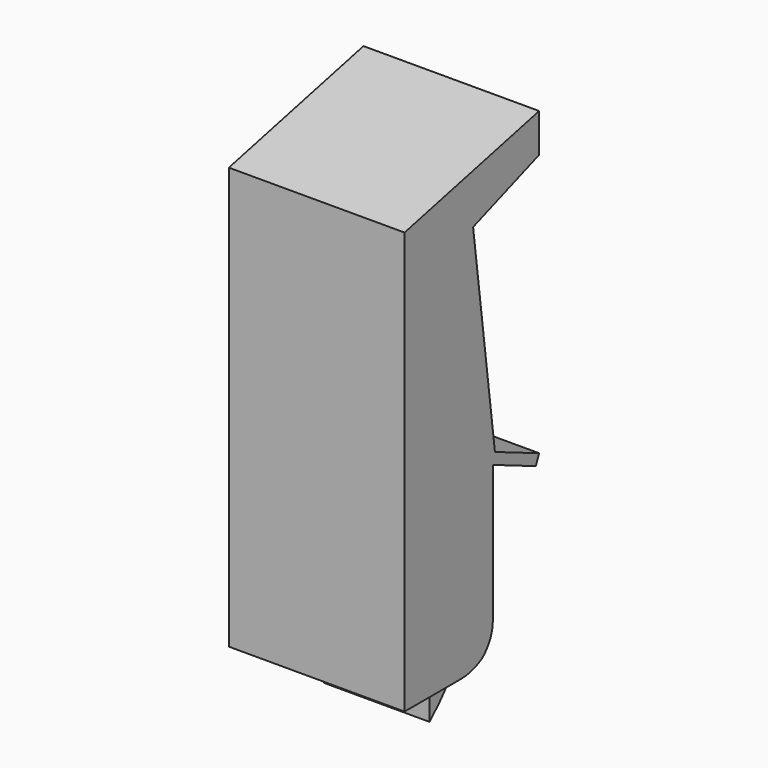
from build123d import *

# Parameters (mm, degrees)
F1_DEPTH     = 500
F2_W         = 500
F2_H         = 299.909304566
F3_DEPTH     = 213.9956919492
F4_W         = 30
F4_H         = 424.5749488473
F5_DEPTH     = 100
F6_DEPTH     = 138
F7_R         = 100
F8_W         = 70
F8_H         = 424.1601228714
F9_DEPTH     = 135
F10_F1_R     = 149.6812408671
F11_W        = 300
F11_H        = 423.4383900396
F11_H_2      = 146.1387078532
F12_DEPTH    = 198
F13_T1_DEPTH = 2527.0832943561
F14_W        = 455.9908173978
F14_H        = 558.4075003862
F15_DEPTH    = 5


# Not quite as in the source:
# - a fillet or chamfer that OpenCascade refuses, or shapes differently, is made with other operations: its cross-section is extruded or revolved along the edge and cut away or added


with BuildPart() as f1:
    # F0 (on Right) → F1 (new body)
    with BuildSketch(Plane.YZ):
        Polygon((-1006.1864304423, 680.3810487322), (-1006.1864304423, -819.6189512678), (-792.191738493, -819.6189512678), (-792.191738493, 13.2260688636), (-539.2304401761, -94.6422840199), (-527.4629834979, -67.0465060217), (-684.6932624212, 0), (-762.4113425204, 594.9452916241), (-527.4629834979, 680.3810487322), (-527.4629834979, 790.310077366), align=None)
    extrude(amount=F1_DEPTH)

    # F2 (on face) → F3 (cut, through all)
    with BuildSketch(Plane(origin=(0, -792.191738493, 0), x_dir=(-1, 0, 0), z_dir=(0, 1, 0))):
        with Locations((-250, -669.6642989848)):
            Rectangle(F2_W, F2_H)
    extrude(amount=-F3_DEPTH, mode=Mode.SUBTRACT)

    # F4 (on face) → F5 (join)
    with BuildSketch(Plane(origin=(0, -792.191738493, 0), x_dir=(-1, 0, 0), z_dir=(0, 1, 0))):
        with Locations((-15, -307.4221722782)):
            Rectangle(F4_W, F4_H)
        with Locations((-485, -307.4221722782)):
            Rectangle(F4_W, F4_H)
    extrude(amount=F5_DEPTH)

    # F6 (add): faces of the model
    f6_faces = [f1.faces().sort_by_distance(p)[0] for p in [
        (15, -742.191738493, -95.1346978545),
        (485, -742.191738493, -95.1346978545),
    ]]
    extrude(f6_faces, amount=F6_DEPTH)

    # F7
    f7_edges = [f1.edges().sort_by_distance(p)[0] for p in [
        (485, -692.191738, -519.709647),
        (15, -692.191738, -519.709647),
    ]]
    fillet(f7_edges, radius=F7_R)

    # F8 (on face) → F9 (join)
    with BuildSketch(Plane(origin=(0, -792.191738493, 0), x_dir=(-1, 0, 0), z_dir=(0, 1, 0))):
        with Locations((-435, -307.6295852661)):
            Rectangle(F8_W, F8_H)
        with Locations((-65, -307.6295852661)):
            Rectangle(F8_W, F8_H)
    extrude(amount=F9_DEPTH)

    # F10: fillet of radius 149.6812408671 on 2 edges, made by hand

    # F10_f1
    f10_f1_edges = [f1.edges().sort_by_distance(p)[0] for p in [
        (435, -657.191738493, -519.7096467018),
    ]]
    fillet(f10_f1_edges, radius=F10_F1_R)

    # F11 (on face) → F12 (join)
    with BuildSketch(Plane(origin=(0, -792.191738493, 0), x_dir=(-1, 0, 0), z_dir=(0, 1, 0))):
        with Locations((-250, -307.2687188502)):
            Rectangle(F11_W, F11_H)
        with Locations((-250, -592.0572677966)):
            Rectangle(F11_W, F11_H_2)
    extrude(amount=F12_DEPTH)

    # F13: fillet of radius 600 on 1 edges, made by hand

    # F13_s2 → F13_t1 (cut)
    with BuildSketch(Plane.YZ.offset(-1013.541647178)):
        with BuildLine():
            ThreePointArc((-792.191738493, -665.1266217232), (-645.9217320181, -463.431114991), (-594.191738493, -219.709962852))
            Line((-594.191738493, -219.709962852), (-594.191738493, -665.1266217232))
            Line((-594.191738493, -665.1266217232), (-792.191738493, -665.1266217232))
        make_face()
    extrude(amount=F13_T1_DEPTH, mode=Mode.SUBTRACT)

    # F14 (on face) → F15 (cut)
    with BuildSketch(Plane(origin=(0, -673.2054408747, -87.9412529416), x_dir=(-1, 0, 0), z_dir=(0, 0.991575486, 0.1295301335))):
        with Locations((-247.8018868715, 387.0010599494)):
            Rectangle(F14_W, F14_H)
    extrude(amount=-F15_DEPTH, mode=Mode.SUBTRACT)


solid = f1.part
